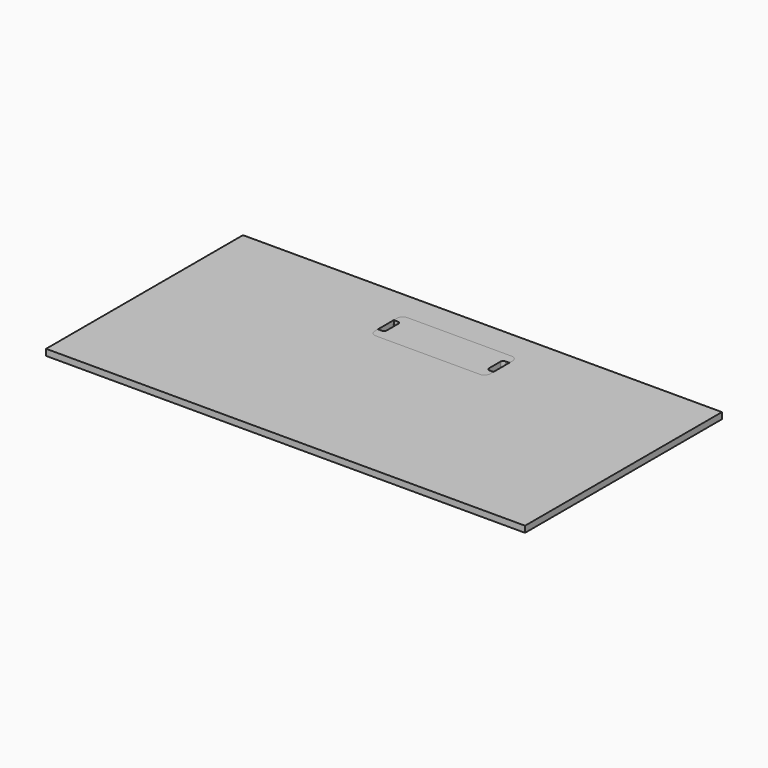
from build123d import *

# Parameters (mm, degrees)
F1_DEPTH  = 19.05
F3_DEPTH  = 19.051
F4_W      = 406.4
F4_H      = 177.8
F5_DEPTH  = 6
F6_W      = 1450
F6_H      = 745
F7_DEPTH  = 19.05
F9_DEPTH  = 12
F11_DEPTH = 7.051
F12_W     = 9.3
F12_H     = 60
F13_DEPTH = 7.051
F14_R     = 3.5


with BuildPart() as f1:
    # F0 (on Top) → F1 (new body)
    with BuildSketch(Plane.XY):
        with BuildLine():
            ThreePointArc((-174.8, -42.8), (-169.8208152802, -54.8208152802), (-157.8, -59.8))
            Line((-157.8, -59.8), (157.8, -59.8))
            ThreePointArc((157.8, -59.8), (169.8208152802, -54.8208152802), (174.8, -42.8))
            Line((174.8, -42.8), (174.8, 42.8))
            ThreePointArc((174.8, 42.8), (169.8208152802, 54.8208152802), (157.8, 59.8))
            Line((157.8, 59.8), (-157.8, 59.8))
            ThreePointArc((-157.8, 59.8), (-169.8208152802, 54.8208152802), (-174.8, 42.8))
            Line((-174.8, 42.8), (-174.8, -42.8))
        make_face()
    extrude(amount=F1_DEPTH)

    # F2 (on face) → F3 (cut, through all)
    with BuildSketch(Plane.XY.offset(19.05)):
        with BuildLine():
            Line((-174.8, 30), (-174.8, -30))
            Line((-174.8, -30), (-163.3, -30))
            ThreePointArc((-163.3, -30), (-157.2895923599, -27.5104076401), (-154.8, -21.5))
            Line((-154.8, -21.5), (-154.8, 21.5))
            ThreePointArc((-154.8, 21.5), (-157.2895923599, 27.5104076401), (-163.3, 30))
            Line((-163.3, 30), (-174.8, 30))
        make_face()
        with BuildLine():
            Line((174.8, -30), (174.8, 30))
            Line((174.8, 30), (163.3, 30))
            ThreePointArc((163.3, 30), (157.2895923599, 27.5104076401), (154.8, 21.5))
            Line((154.8, 21.5), (154.8, -21.5))
            ThreePointArc((154.8, -21.5), (157.2895923599, -27.5104076401), (163.3, -30))
            Line((163.3, -30), (174.8, -30))
        make_face()
    extrude(amount=-F3_DEPTH, mode=Mode.SUBTRACT)

    # F4 (on face) → F5 (cut)
    with BuildSketch(Plane(origin=(0, 0, 0), x_dir=(1, 0, 0), z_dir=(0, 0, -1))):
        Rectangle(F4_W, F4_H)
        with BuildLine():
            ThreePointArc((161.5, -42.8), (160.4162950904, -45.4162950904), (157.8, -46.5))
            Line((157.8, -46.5), (-157.8, -46.5))
            ThreePointArc((-157.8, -46.5), (-160.4162950904, -45.4162950904), (-161.5, -42.8))
            Line((-161.5, -42.8), (-161.5, 42.8))
            ThreePointArc((-161.5, 42.8), (-160.4162950904, 45.4162950904), (-157.8, 46.5))
            Line((-157.8, 46.5), (157.8, 46.5))
            ThreePointArc((157.8, 46.5), (160.4162950904, 45.4162950904), (161.5, 42.8))
            Line((161.5, 42.8), (161.5, -42.8))
        make_face(mode=Mode.SUBTRACT)
    extrude(amount=-F5_DEPTH, mode=Mode.SUBTRACT)


with BuildPart() as f7:
    # F6 (on face) → F7 (new body)
    with BuildSketch(Plane.XY.offset(19.05)):
        with Locations((0, -225.7)):
            Rectangle(F6_W, F6_H)
    extrude(amount=-F7_DEPTH)

    # F8 (on face) → F9 (cut)
    with BuildSketch(Plane.XY.offset(19.05)):
        with BuildLine():
            Line((157.8, 59.8), (-157.8, 59.8))
            ThreePointArc((-157.8, 59.8), (-169.8208152802, 54.8208152802), (-174.8, 42.8))
            Line((-174.8, 42.8), (-174.8, 30))
            Line((-174.8, 30), (-174.8, -30))
            Line((-174.8, -30), (-174.8, -42.8))
            ThreePointArc((-174.8, -42.8), (-169.8208152802, -54.8208152802), (-157.8, -59.8))
            Line((-157.8, -59.8), (157.8, -59.8))
            ThreePointArc((157.8, -59.8), (169.8208152802, -54.8208152802), (174.8, -42.8))
            Line((174.8, -42.8), (174.8, -30))
            Line((174.8, -30), (174.8, 30))
            Line((174.8, 30), (174.8, 42.8))
            ThreePointArc((174.8, 42.8), (169.8208152802, 54.8208152802), (157.8, 59.8))
        make_face()
    extrude(amount=-F9_DEPTH, mode=Mode.SUBTRACT)

    # F10 (on face) → F11 (cut, through all)
    with BuildSketch(Plane.XY.offset(7.05)):
        with BuildLine():
            Line((-165.5, -30), (-165.5, -42.8))
            ThreePointArc((-165.5, -42.8), (-163.2447222151, -48.2447222151), (-157.8, -50.5))
            Line((-157.8, -50.5), (157.8, -50.5))
            ThreePointArc((157.8, -50.5), (163.2447222151, -48.2447222151), (165.5, -42.8))
            Line((165.5, -42.8), (165.5, -30))
            Line((165.5, -30), (165.5, 30))
            Line((165.5, 30), (165.5, 42.8))
            ThreePointArc((165.5, 42.8), (163.2447222151, 48.2447222151), (157.8, 50.5))
            Line((157.8, 50.5), (-157.8, 50.5))
            ThreePointArc((-157.8, 50.5), (-163.2447222151, 48.2447222151), (-165.5, 42.8))
            Line((-165.5, 42.8), (-165.5, 30))
            Line((-165.5, 30), (-165.5, -30))
        make_face()
    extrude(amount=-F11_DEPTH, mode=Mode.SUBTRACT)

    # F12 (on face) → F13 (cut, through all)
    with BuildSketch(Plane.XY.offset(7.05)):
        with Locations((-170.15, 0)):
            Rectangle(F12_W, F12_H)
        with Locations((170.15, 0)):
            Rectangle(F12_W, F12_H)
    extrude(amount=-F13_DEPTH, mode=Mode.SUBTRACT)

    # F14
    f14_edges = [f7.edges().sort_by_distance(p)[0] for p in [
        (-165.5, 30, 3.525),
        (-174.8, 30, 3.525),
        (-174.8, -30, 3.525),
        (-165.5, -30, 3.525),
        (165.5, 30, 3.525),
        (174.8, 30, 3.525),
        (165.5, -30, 3.525),
        (174.8, -30, 3.525),
    ]]
    fillet(f14_edges, radius=F14_R)


solid = Compound([f1.part, f7.part])
